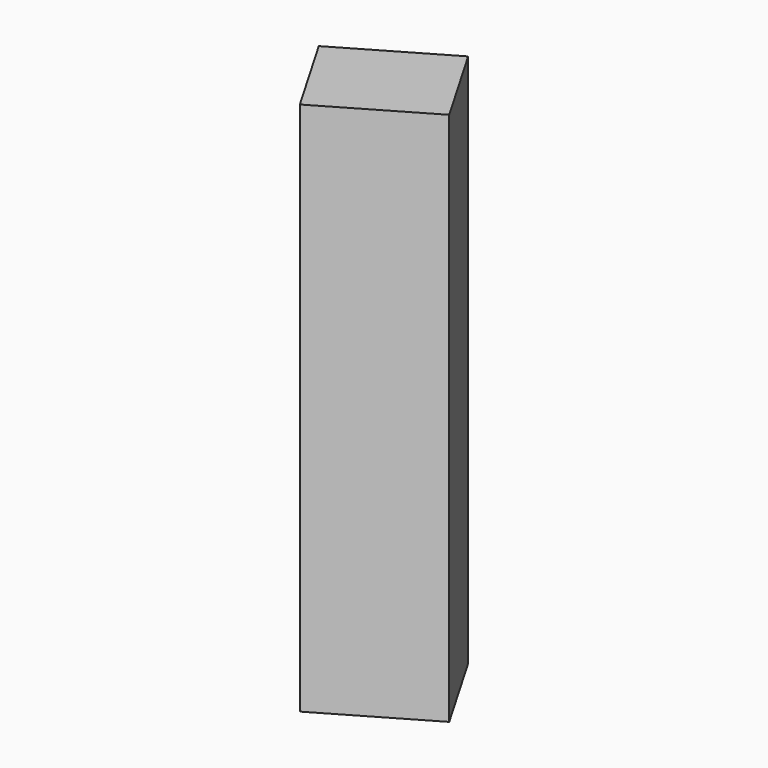
from build123d import *

# Parameters (mm, degrees)
F1_E2_W  = 21.512664049
F1_E2_H  = 115.1049882174
F3_DEPTH = 25.4
F4_T     = -1.524


with BuildPart() as f3:
    # F1_E2 (on explicit) → F3 (new body)
    with BuildSketch(Plane(origin=(0, 54.6783059835, 0), x_dir=(-0.5023234046, 0.8646798235, 0), z_dir=(0.8646798235, 0.5023234046, 0))):
        with Locations((10.7563320245, 57.5524941087)):
            Rectangle(F1_E2_W, F1_E2_H)
    extrude(amount=F3_DEPTH)

    # F4
    f4_openings = [f3.faces().sort_by_distance(p)[0] for p in [
        (5.578276, 70.358596, 0),
    ]]
    offset(amount=F4_T, openings=f4_openings)


solid = f3.part
